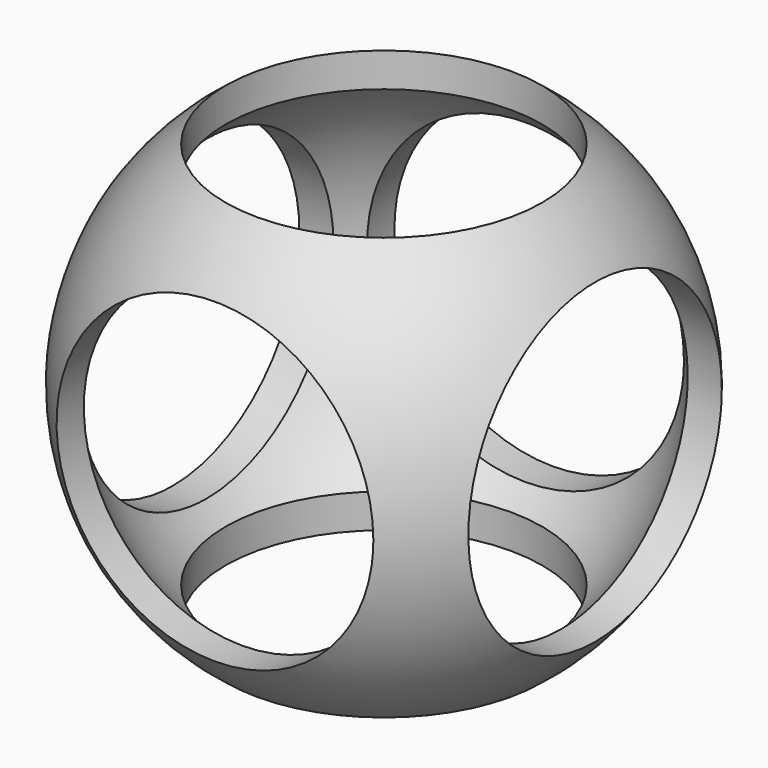
from build123d import *

# Parameters (mm, degrees)
F2_R          = 30
F3_DEPTH      = 50.001
F3_DEPTH_BACK = 50.001
F4_R          = 30
F5_DEPTH      = 50.001
F5_DEPTH_BACK = 50.001
F6_R          = 30
F7_DEPTH      = 50.001
F7_DEPTH_BACK = 50.001


# Not quite as in the source:
# - a feature names something its author has since deleted; it is built from what else it names


with BuildPart() as f1:
    # F0 (on Front) → F1 (revolve)
    with BuildSketch(Plane.XZ):
        with BuildLine():
            Line((0, -50), (0, 0))
            Line((0, 0), (0, 50))
            ThreePointArc((0, 50), (-50, 0), (0, -50))
        make_face()
    revolve(axis=Axis((0, 0, 25), (0, 0, 1)))

    # F2 (on Front) → F3 (cut, two sides)
    with BuildSketch(Plane.XZ) as f3_sk:
        Circle(F2_R)
    extrude(amount=-F3_DEPTH, mode=Mode.SUBTRACT)
    extrude(f3_sk.sketch, amount=F3_DEPTH_BACK, mode=Mode.SUBTRACT)

    # F4 (on Right) → F5 (cut, two sides)
    with BuildSketch(Plane.YZ) as f5_sk:
        Circle(F4_R)
    extrude(amount=-F5_DEPTH, mode=Mode.SUBTRACT)
    extrude(f5_sk.sketch, amount=F5_DEPTH_BACK, mode=Mode.SUBTRACT)

    # F6 (on Top) → F7 (cut, two sides)
    with BuildSketch(Plane.XY) as f7_sk:
        Circle(F6_R)
    extrude(amount=F7_DEPTH, mode=Mode.SUBTRACT)
    extrude(f7_sk.sketch, amount=-F7_DEPTH_BACK, mode=Mode.SUBTRACT)

    # F8 (on Front) → F9 (revolve, cut)
    with BuildSketch(Plane.XZ):
        with BuildLine():
            Line((0, -45), (0, 0))
            Line((0, 0), (0, 45))
            ThreePointArc((0, 45), (-45, 0), (0, -45))
        make_face()
    revolve(axis=Axis((0, 0, 22.5), (0, 0, 1)), mode=Mode.SUBTRACT)


solid = f1.part
